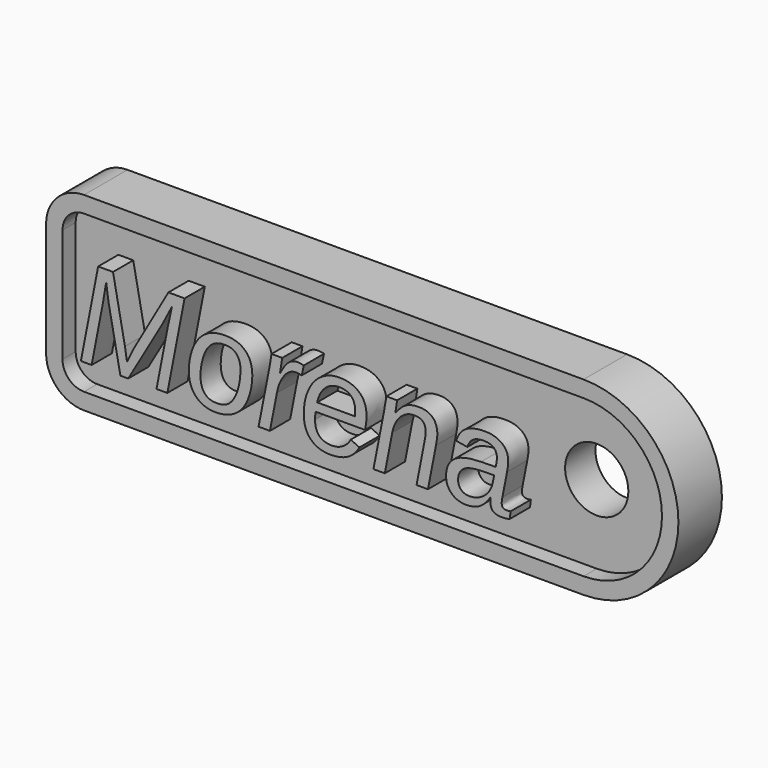
from build123d import *

# Parameters (mm, degrees)
F0_R         = 2.5
F1_DEPTH     = 3
F2_TEXT_SIZE = 10.2171136654
F3_DEPTH     = 2
F5_DEPTH     = 1.3


# Not quite as in the source:
# - Text() gives the source's letters only with a copy of the font that has no kerning and outlines rounded to 1/6400 em; it was checked with that copy


with BuildPart() as f1:
    # F0 (on Front) → F1 (new body)
    with BuildSketch(Plane.XZ):
        with BuildLine():
            Line((21.25, 7.5), (-18.25, 7.5))
            ThreePointArc((-18.25, 7.5), (-20.3713203436, 6.6213203436), (-21.25, 4.5))
            Line((-21.25, 4.5), (-21.25, -4.5))
            ThreePointArc((-21.25, -4.5), (-20.3713203436, -6.6213203436), (-18.25, -7.5))
            Line((-18.25, -7.5), (21.25, -7.5))
            ThreePointArc((21.25, -7.5), (28.75, 0), (21.25, 7.5))
        make_face()
        with Locations((21.25, 0)):
            Circle(F0_R, mode=Mode.SUBTRACT)
    extrude(amount=F1_DEPTH)

    # F2 (on face) → F3 (join)
    with BuildSketch(Plane.XZ.offset(3)):
        with Locations((-18.25, -3.6781609195)):
            Text('Morena', F2_TEXT_SIZE, font='Arimo', font_style=FontStyle.ITALIC, text_align=(TextAlign.LEFT, TextAlign.BOTTOM))
    extrude(amount=F3_DEPTH)

    # F4 (on face) → F5 (join)
    with BuildSketch(Plane.XZ.offset(3)):
        with BuildLine():
            ThreePointArc((21.25, -7.5), (28.75, 0), (21.25, 7.5))
            Line((21.25, 7.5), (-18.25, 7.5))
            ThreePointArc((-18.25, 7.5), (-20.3713203436, 6.6213203436), (-21.25, 4.5))
            Line((-21.25, 4.5), (-21.25, -4.5))
            ThreePointArc((-21.25, -4.5), (-20.3713203436, -6.6213203436), (-18.25, -7.5))
            Line((-18.25, -7.5), (21.25, -7.5))
        make_face()
        with BuildLine():
            ThreePointArc((-19.95, 4.5), (-19.452081528, 5.702081528), (-18.25, 6.2))
            Line((-18.25, 6.2), (21.25, 6.2))
            ThreePointArc((21.25, 6.2), (27.45, 0), (21.25, -6.2))
            Line((21.25, -6.2), (-18.25, -6.2))
            ThreePointArc((-18.25, -6.2), (-19.452081528, -5.702081528), (-19.95, -4.5))
            Line((-19.95, -4.5), (-19.95, 4.5))
        make_face(mode=Mode.SUBTRACT)
    extrude(amount=F5_DEPTH)


solid = f1.part
